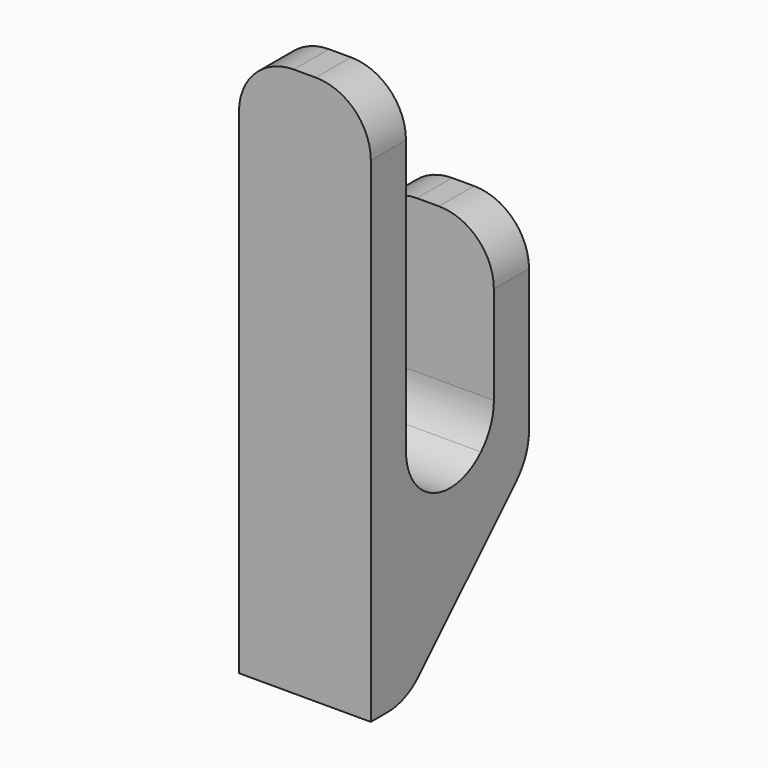
from build123d import *

# Parameters (mm, degrees)
F0_W     = 6
F0_H     = 50
F1_DEPTH = 4
F3_DEPTH = 12
F4_R     = 4.99999
F5_R     = 5


# Not quite as in the source:
# - a fillet or chamfer is up to 0.001 mm smaller than in the source, because OpenCascade refuses the exact size


with BuildPart() as f1:
    # F0 (on Front) → F1 (new body)
    with BuildSketch(Plane.XZ):
        with Locations((9, 25)):
            Rectangle(F0_W, F0_H)
        with Locations((3, 25)):
            Rectangle(F0_W, F0_H)
    extrude(amount=F1_DEPTH)

    # F2 (on Right) → F3 (join)
    with BuildSketch(Plane.YZ):
        Polygon((0, 8), (0, 0), (14, 14), (14, 34), (10, 34), (10, 18), align=None)
    extrude(amount=F3_DEPTH)

    # F4 (radius 5 in the source; OpenCascade refuses exactly that, so slightly less here)
    f4_edges = [f1.edges().sort_by_distance(p)[0] for p in [
        (0, -2, 50),
        (12, -2, 50),
        (0, 12, 34),
        (12, 12, 34),
        (6, 10, 18),
        (6, 14, 14),
        (6, 0, 8),
    ]]
    fillet(f4_edges, radius=F4_R)

    # F5
    f5_edges = [f1.edges().sort_by_distance(p)[0] for p in [
        (6, 0, 0),
    ]]
    fillet(f5_edges, radius=F5_R)


solid = f1.part
